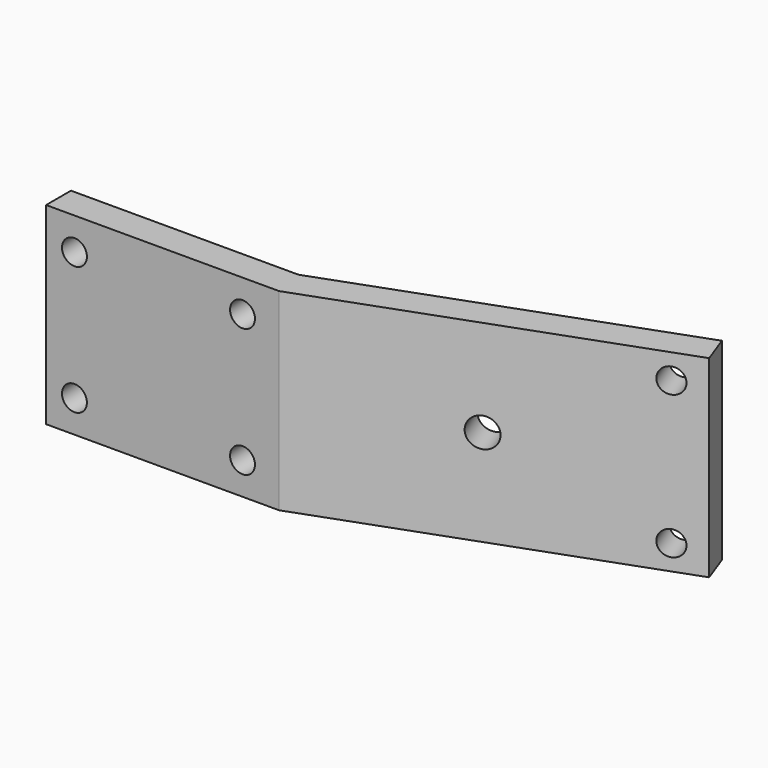
from build123d import *

# Parameters (mm, degrees)
F1_W     = 10
F1_H     = 62
F4_D     = 8
F5_D     = 9.525
F7_D     = 8
F8_ANGLE = -20


# Not quite as in the source:
# - a length typed as a fraction of an inch, garbled in the dataset ("3 / 203.2 mm" for 3/8 in), is restored


with BuildPart() as f2:
    # F2: sweep along a path in F0
    with BuildLine(Plane.XY) as f2_path:
        Line((0, 0), (-113, 0))
        Line((-113, 0), (-182.5372539382, 25.3094906061))
    # F1 (on Right) → F2 (sweep)
    with BuildSketch(Plane.YZ):
        Rectangle(F1_W, F1_H)
    sweep(path=f2_path.line, transition=Transition.RIGHT)

    # F4 (through all)
    with Locations(Plane(origin=(0, 5, 0), x_dir=(-1, 0, 0), z_dir=(0, 1, 0))):
        with Locations((10, -23), (10, 23)):
            Hole(F4_D / 2)

    # F5 (through all)
    with Locations(Plane(origin=(0, 5, 0), x_dir=(-1, 0, 0), z_dir=(0, 1, 0))):
        with Locations((60, 0)):
            Hole(F5_D / 2)

    # F7 (through all)
    with Locations(Plane(origin=(-11.5083882471, -31.6190368434, 0), x_dir=(-0.9396926208, 0.3420201433, 0), z_dir=(0.3420201433, 0.9396926208, 0))):
        with Locations((117.0669010524, 20.6375), (171.0669010524, 20.6375), (171.0669010524, -20.6375), (117.0669010524, -20.6375)):
            Hole(F7_D / 2)


with BuildPart() as f2_1:
    # F8: moved
    add(f2.part.rotate(Axis((-184.2473546548, 20.6110275022, 0), (0, 0, -1)), F8_ANGLE))


solid = f2_1.part
